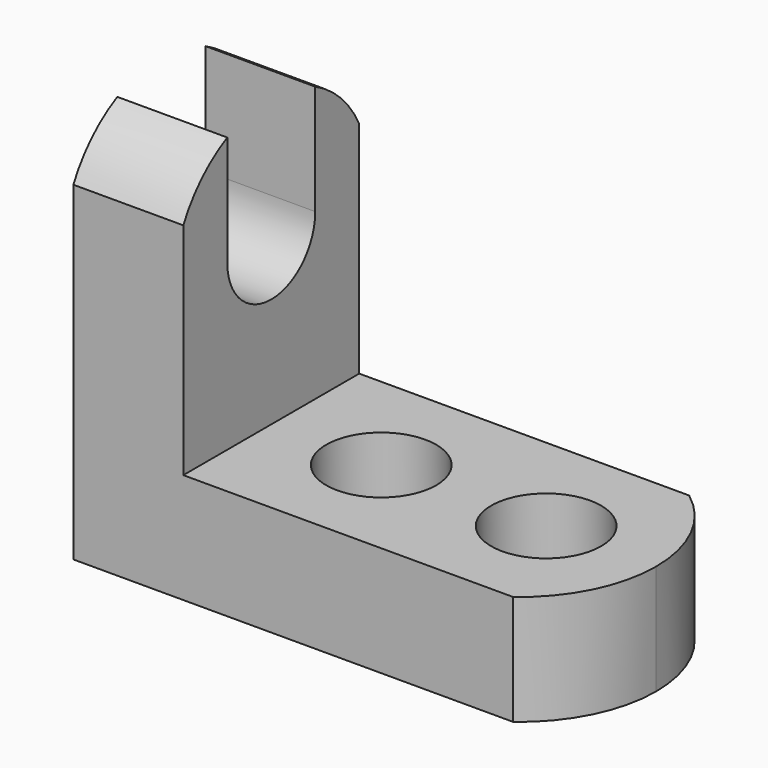
from build123d import *

# Parameters (mm, degrees)
F0_W      = 57.15
F0_H      = 44.45
F1_DEPTH  = 25.4
F2_W      = 44.45
F2_H      = 31.75
F3_DEPTH  = 25.401
F5_DEPTH  = 12.701
F6_R      = 6.35
F7_DEPTH  = 12.701
F9_DEPTH  = 12.701
F11_DEPTH = 12.701


with BuildPart() as f1:
    # F0 (on Front) → F1 (new body)
    with BuildSketch(Plane.XZ):
        with Locations((-28.575, 22.225)):
            Rectangle(F0_W, F0_H)
    extrude(amount=F1_DEPTH)

    # F2 (on face) → F3 (cut, through all)
    with BuildSketch(Plane.XZ.offset(25.4)):
        with Locations((-22.225, 28.575)):
            Rectangle(F2_W, F2_H)
    extrude(amount=-F3_DEPTH, mode=Mode.SUBTRACT)

    # F4 (on face) → F5 (cut, through all)
    with BuildSketch(Plane.XY.offset(12.7)):
        with BuildLine():
            Line((0, -12.7), (0, 0))
            Line((0, 0), (-6.35, 0))
            ThreePointArc((-6.35, 0), (-1.6759683429, -5.6004841714), (0, -12.7))
        make_face()
        with BuildLine():
            Line((0, -25.4), (0, -12.7))
            ThreePointArc((0, -12.7), (-1.6759683429, -19.7995158286), (-6.35, -25.4))
            Line((-6.35, -25.4), (0, -25.4))
        make_face()
    extrude(amount=-F5_DEPTH, mode=Mode.SUBTRACT)

    # F6 (on face) → F7 (cut, through all)
    with BuildSketch(Plane.XY.offset(12.7)):
        with Locations((-31.75, -12.7)):
            Circle(F6_R)
        with Locations((-12.7, -12.7)):
            Circle(F6_R)
    extrude(amount=-F7_DEPTH, mode=Mode.SUBTRACT)

    # F8 (on face) → F9 (cut, through all)
    with BuildSketch(Plane.YZ.offset(-44.45)):
        with BuildLine():
            ThreePointArc((-19.05, 31.75), (-12.7, 38.1), (-6.35, 31.75))
            Line((-6.35, 31.75), (-6.35, 44.45))
            Line((-6.35, 44.45), (-19.05, 44.45))
            Line((-19.05, 44.45), (-19.05, 31.75))
        make_face()
        with BuildLine():
            ThreePointArc((-19.05, 31.75), (-12.7, 25.4), (-6.35, 31.75))
            ThreePointArc((-6.35, 31.75), (-12.7, 38.1), (-19.05, 31.75))
        make_face()
    extrude(amount=-F9_DEPTH, mode=Mode.SUBTRACT)

    # F10 (on face) → F11 (cut, through all)
    with BuildSketch(Plane.YZ.offset(-44.45)):
        with BuildLine():
            Line((-19.05, 44.45), (-25.4, 44.45))
            Line((-25.4, 44.45), (-25.4, 38.1))
            ThreePointArc((-25.4, 38.1), (-22.740231571, 41.790231571), (-19.05, 44.45))
        make_face()
        with BuildLine():
            Line((0, 44.45), (-6.35, 44.45))
            ThreePointArc((-6.35, 44.45), (-2.659768429, 41.790231571), (0, 38.1))
            Line((0, 38.1), (0, 44.45))
        make_face()
    extrude(amount=-F11_DEPTH, mode=Mode.SUBTRACT)


solid = f1.part
